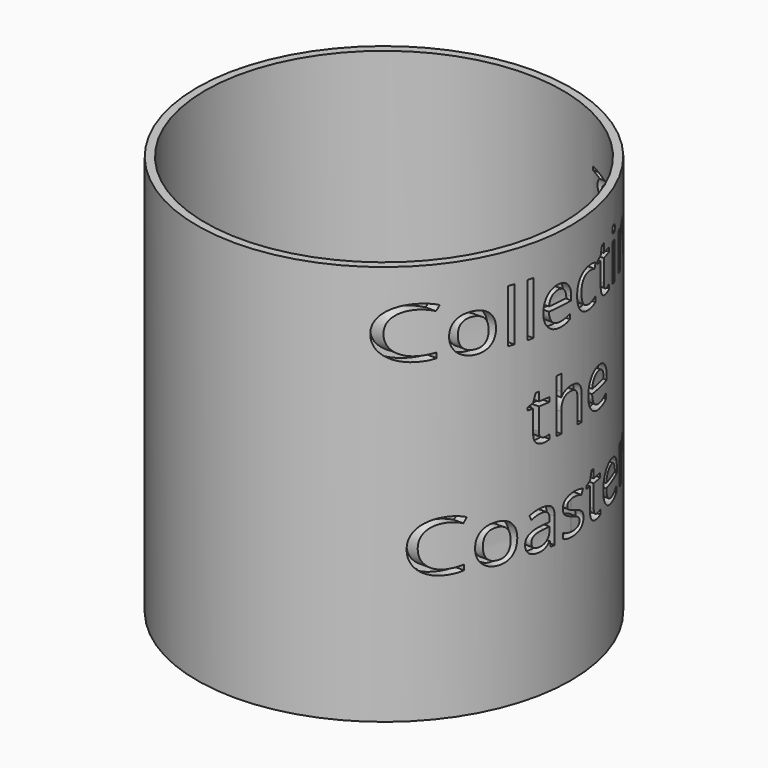
from build123d import *

# Parameters (mm, degrees)
F0_R         = 35
F1_DEPTH     = 75
F2_R         = 33.5
F3_DEPTH     = 70
F4_TEXT_SIZE = 6.1913514559
F5_DEPTH     = 5.001
F6_TEXT_SIZE = 13.081692444
F7_DEPTH     = 35.0010001


# Not quite as in the source:
# - Text() gives the source's letters only with a copy of the font that has no kerning and outlines rounded to 1/6400 em; it was checked with that copy


with BuildPart() as f1:
    # F0 (on Top) → F1 (new body)
    with BuildSketch(Plane.XY):
        Circle(F0_R)
    extrude(amount=F1_DEPTH)

    # F2 (on face) → F3 (cut)
    with BuildSketch(Plane.XY.offset(75)):
        Circle(F2_R)
    extrude(amount=-F3_DEPTH, mode=Mode.SUBTRACT)

    # F4 (on face) → F5 (cut, through all)
    with BuildSketch(Plane.XY.offset(5)):
        with Locations((-13.1988143722, 10.2983738504)):
            Text('Prof Stols', F4_TEXT_SIZE, font='Open Sans', text_align=(TextAlign.LEFT, TextAlign.BOTTOM))
        with Locations((-24.4603022313, 1.8781358704)):
            Text('Keeping together', F4_TEXT_SIZE, font='Open Sans', text_align=(TextAlign.LEFT, TextAlign.BOTTOM))
        with Locations((-3.5461104929, -6.5421021097)):
            Text('the', F4_TEXT_SIZE, font='Open Sans', text_align=(TextAlign.LEFT, TextAlign.BOTTOM))
        with Locations((-14.8075983521, -14.9623400898)):
            Text('Coasters', F4_TEXT_SIZE, font='Open Sans', text_align=(TextAlign.LEFT, TextAlign.BOTTOM))
    extrude(amount=-F5_DEPTH, mode=Mode.SUBTRACT)

    # F6 (on Right) → F7 (cut, through all)
    with BuildSketch(Plane.YZ):
        with Locations((-29.3385478663, 59.29740543)):
            Text('Collecting', F6_TEXT_SIZE, font='Open Sans', text_align=(TextAlign.LEFT, TextAlign.BOTTOM))
        with Locations((-8.9433717404, 41.5063037062)):
            Text('the', F6_TEXT_SIZE, font='Open Sans', text_align=(TextAlign.LEFT, TextAlign.BOTTOM))
        with Locations((-25.9393518453, 23.7152019824)):
            Text('Coasters', F6_TEXT_SIZE, font='Open Sans', text_align=(TextAlign.LEFT, TextAlign.BOTTOM))
    extrude(amount=F7_DEPTH, mode=Mode.SUBTRACT)


solid = f1.part
